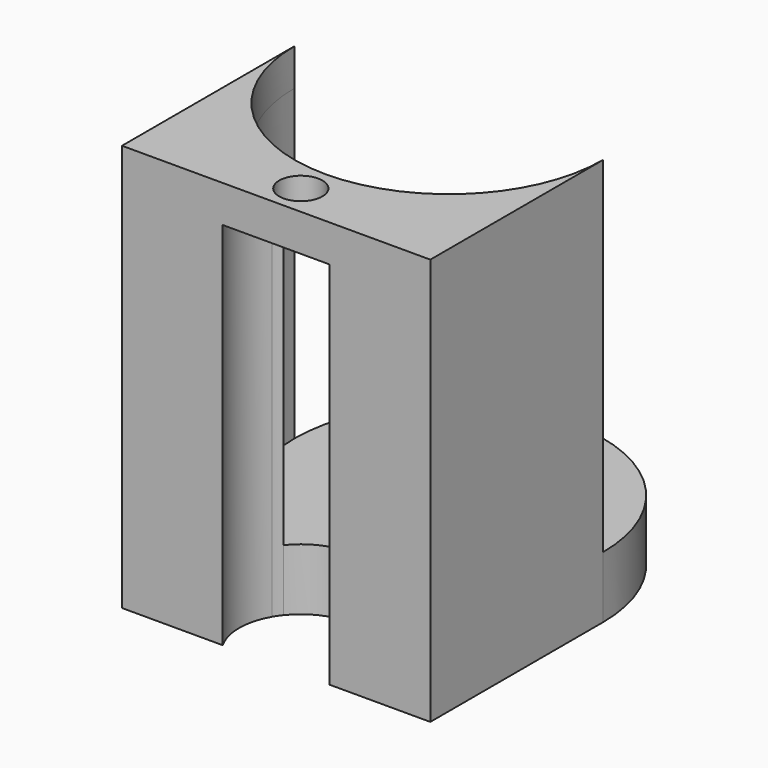
from build123d import *

# Parameters (mm, degrees)
F1_DEPTH = 5
F2_DEPTH = 30
F3_R     = 1.75
F4_DEPTH = 3


with BuildPart() as f1:
    # F0 (on Top) → F1 (new body)
    with BuildSketch(Plane.XY):
        with BuildLine():
            Line((6.25, 0), (10, 0))
            ThreePointArc((10, 0), (0, 10), (-10, 0))
            Line((-10, 0), (-6.25, 0))
            ThreePointArc((-6.25, 0), (0, 6.25), (6.25, 0))
        make_face()
        with BuildLine():
            Line((12.5, 0), (10, 0))
            ThreePointArc((10, 0), (8.7372269275, -4.8642435813), (5.2678268764, -8.5))
            Line((5.2678268764, -8.5), (9.1651513899, -8.5))
            ThreePointArc((9.1651513899, -8.5), (11.6364597789, -4.5653919671), (12.5, 0))
        make_face()
        with BuildLine():
            ThreePointArc((5.2678268764, -8.5), (8.7372269275, -4.8642435813), (10, 0))
            Line((10, 0), (6.25, 0))
            ThreePointArc((6.25, 0), (0, -6.25), (-6.25, 0))
            Line((-6.25, 0), (-10, 0))
            ThreePointArc((-10, 0), (-8.7372269275, -4.8642435813), (-5.2678268764, -8.5))
            Line((-5.2678268764, -8.5), (5.2678268764, -8.5))
        make_face()
        with BuildLine():
            ThreePointArc((-10, 0), (0, 10), (10, 0))
            Line((10, 0), (12.5, 0))
            ThreePointArc((12.5, 0), (0, 12.5), (-12.5, 0))
            Line((-12.5, 0), (-10, 0))
        make_face()
        with BuildLine():
            ThreePointArc((-5.2678268764, -8.5), (-8.7372269275, -4.8642435813), (-10, 0))
            Line((-10, 0), (-12.5, 0))
            ThreePointArc((-12.5, 0), (-11.6364597789, -4.5653919671), (-9.1651513899, -8.5))
            Line((-9.1651513899, -8.5), (-5.2678268764, -8.5))
        make_face()
        with BuildLine():
            Line((9.1651513899, -8.5), (5.2678268764, -8.5))
            ThreePointArc((5.2678268764, -8.5), (2.7386127875, -9.6176920308), (0, -10))
            ThreePointArc((0, -10), (2.1650635095, -10.4930609057), (3.903123749, -11.875))
            ThreePointArc((3.903123749, -11.875), (6.7485265078, -10.5217579317), (9.1651513899, -8.5))
        make_face()
        with BuildLine():
            ThreePointArc((0, -10), (2.7386127875, -9.6176920308), (5.2678268764, -8.5))
            Line((5.2678268764, -8.5), (-5.2678268764, -8.5))
            ThreePointArc((-5.2678268764, -8.5), (-2.7386127875, -9.6176920308), (0, -10))
        make_face()
        with BuildLine():
            ThreePointArc((0, -10), (-2.7386127875, -9.6176920308), (-5.2678268764, -8.5))
            Line((-5.2678268764, -8.5), (-9.1651513899, -8.5))
            ThreePointArc((-9.1651513899, -8.5), (-6.7485265078, -10.5217579317), (-3.903123749, -11.875))
            ThreePointArc((-3.903123749, -11.875), (-2.1650635095, -10.4930609057), (0, -10))
        make_face()
    extrude(amount=F1_DEPTH)

    # F0 (on Top) → F2 (join)
    with BuildSketch(Plane.XY):
        with BuildLine():
            ThreePointArc((-9.1651513899, -8.5), (-11.6364597789, -4.5653919671), (-12.5, 0))
            Line((-12.5, 0), (-12.5, -8.5))
            Line((-12.5, -8.5), (-9.1651513899, -8.5))
        make_face()
        with BuildLine():
            Line((12.5, -8.5), (12.5, 0))
            ThreePointArc((12.5, 0), (11.6364597789, -4.5653919671), (9.1651513899, -8.5))
            Line((9.1651513899, -8.5), (12.5, -8.5))
        make_face()
        with BuildLine():
            Line((12.5, -8.5), (9.1651513899, -8.5))
            ThreePointArc((9.1651513899, -8.5), (6.7485265078, -10.5217579317), (3.903123749, -11.875))
            ThreePointArc((3.903123749, -11.875), (4.1284695472, -12.1794080057), (4.3301270189, -12.5))
            Line((4.3301270189, -12.5), (12.5, -12.5))
            Line((12.5, -12.5), (12.5, -8.5))
        make_face()
        with BuildLine():
            ThreePointArc((-3.903123749, -11.875), (-6.7485265078, -10.5217579317), (-9.1651513899, -8.5))
            Line((-9.1651513899, -8.5), (-12.5, -8.5))
            Line((-12.5, -8.5), (-12.5, -12.5))
            Line((-12.5, -12.5), (-4.3301270189, -12.5))
            ThreePointArc((-4.3301270189, -12.5), (-4.1284695472, -12.1794080057), (-3.903123749, -11.875))
        make_face()
        with BuildLine():
            Line((-4.3301270189, -12.5), (-12.5, -12.5))
            Line((-12.5, -12.5), (-12.5, -17.5))
            Line((-12.5, -17.5), (-4.3301270189, -17.5))
            ThreePointArc((-4.3301270189, -17.5), (-5, -15), (-4.3301270189, -12.5))
        make_face()
        with BuildLine():
            Line((12.5, -17.5), (12.5, -12.5))
            Line((12.5, -12.5), (4.3301270189, -12.5))
            ThreePointArc((4.3301270189, -12.5), (4.8296291314, -13.7059047745), (5, -15))
            ThreePointArc((5, -15), (4.8296291314, -16.2940952255), (4.3301270189, -17.5))
            Line((4.3301270189, -17.5), (12.5, -17.5))
        make_face()
    extrude(amount=F2_DEPTH)

    # F3 (on face) → F4 (join)
    with BuildSketch(Plane.XY.offset(30)):
        with BuildLine():
            Line((0, -12.5), (-4.3301270189, -12.5))
            ThreePointArc((-4.3301270189, -12.5), (-5, -15), (-4.3301270189, -17.5))
            Line((-4.3301270189, -17.5), (12.5, -17.5))
            Line((12.5, -17.5), (12.5, -12.5))
            Line((12.5, -12.5), (0, -12.5))
        make_face()
        with Locations((0, -15)):
            Circle(F3_R, mode=Mode.SUBTRACT)
        with BuildLine():
            ThreePointArc((-3.903123749, -11.875), (-10.1251925133, -7.3301075414), (-12.5, 0))
            Line((-12.5, 0), (-12.5, -12.5))
            Line((-12.5, -12.5), (-4.3301270189, -12.5))
            ThreePointArc((-4.3301270189, -12.5), (-4.1284695472, -12.1794080057), (-3.903123749, -11.875))
        make_face()
        with BuildLine():
            Line((-4.3301270189, -12.5), (-12.5, -12.5))
            Line((-12.5, -12.5), (-12.5, -17.5))
            Line((-12.5, -17.5), (-4.3301270189, -17.5))
            ThreePointArc((-4.3301270189, -17.5), (-5, -15), (-4.3301270189, -12.5))
        make_face()
        with BuildLine():
            Line((12.5, -12.5), (12.5, 0))
            ThreePointArc((12.5, 0), (8.8388347648, -8.8388347648), (0, -12.5))
            Line((0, -12.5), (12.5, -12.5))
        make_face()
        with BuildLine():
            ThreePointArc((0, -12.5), (-1.9764235376, -12.3427610363), (-3.903123749, -11.875))
            ThreePointArc((-3.903123749, -11.875), (-4.1284695472, -12.1794080057), (-4.3301270189, -12.5))
            Line((-4.3301270189, -12.5), (0, -12.5))
        make_face()
    extrude(amount=F4_DEPTH)


solid = f1.part
